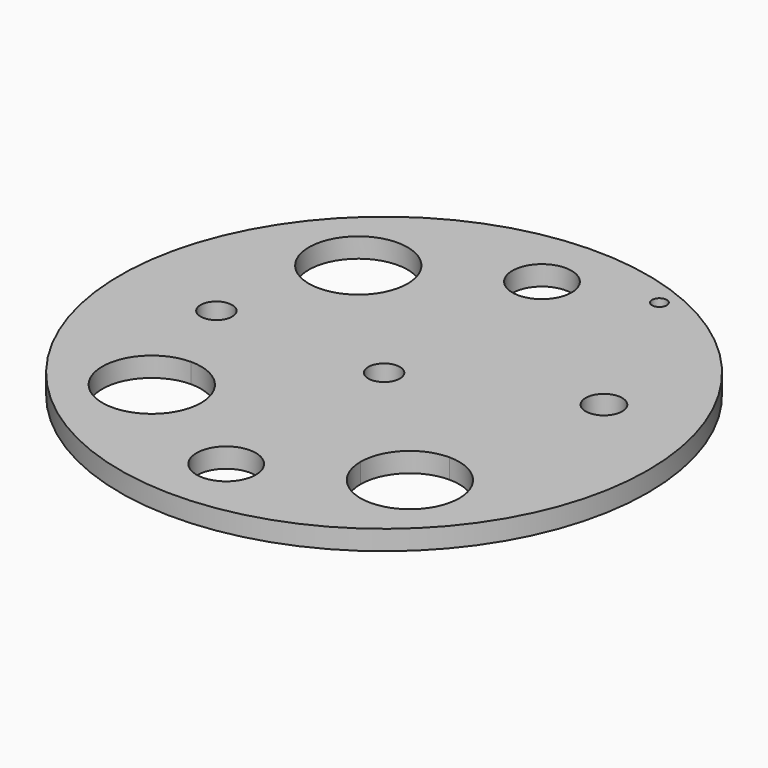
from build123d import *

# Parameters (mm, degrees)
F0_R     = 26.75
F0_R_2   = 3
F0_R_3   = 1.6
F0_R_4   = 1.85
F0_R_5   = 0.75
F1_DEPTH = 2


# Not quite as in the source:
# - a feature names something its author has since deleted; it is built from what else it names


with BuildPart() as f1:
    # F0 (on Top) → F1 (new body)
    with BuildSketch(Plane.XY):
        Circle(F0_R)
        with Locations((0, -20)):
            Circle(F0_R_2, mode=Mode.SUBTRACT)
        with Locations((-17, 0)):
            Circle(F0_R_3, mode=Mode.SUBTRACT)
        with BuildLine():
            Line((-8.081475452, 13.081475452), (13.081475452, 13.081475452))
            Line((13.081475452, 13.081475452), (13.081475452, -8.081475452))
            ThreePointArc((13.081475452, -8.081475452), (16.6170093579, -9.545941546), (18.081475452, -13.081475452))
            ThreePointArc((18.081475452, -13.081475452), (13.081475452, -18.081475452), (8.081475452, -13.081475452))
            Line((8.081475452, -13.081475452), (-8.081475452, -13.081475452))
            ThreePointArc((-8.081475452, -13.081475452), (-16.6170093579, -16.6170093579), (-13.081475452, -8.081475452))
            Line((-13.081475452, -8.081475452), (-13.081475452, 8.081475452))
            ThreePointArc((-13.081475452, 8.081475452), (-16.6170093579, 16.6170093579), (-8.081475452, 13.081475452))
        make_face(mode=Mode.SUBTRACT)
        with Locations((0, 20)):
            Circle(F0_R_2, mode=Mode.SUBTRACT)
        with Locations((17, 6.6)):
            Circle(F0_R_4, mode=Mode.SUBTRACT)
        with Locations((9.5, 23)):
            Circle(F0_R_5, mode=Mode.SUBTRACT)
        with BuildLine():
            Line((13.081475452, -8.081475452), (13.081475452, 13.081475452))
            Line((13.081475452, 13.081475452), (-8.081475452, 13.081475452))
            ThreePointArc((-8.081475452, 13.081475452), (-9.545941546, 9.545941546), (-13.081475452, 8.081475452))
            Line((-13.081475452, 8.081475452), (-13.081475452, -8.081475452))
            ThreePointArc((-13.081475452, -8.081475452), (-9.545941546, -9.545941546), (-8.081475452, -13.081475452))
            Line((-8.081475452, -13.081475452), (8.081475452, -13.081475452))
            ThreePointArc((8.081475452, -13.081475452), (9.545941546, -9.545941546), (13.081475452, -8.081475452))
        make_face()
        Circle(F0_R_3, mode=Mode.SUBTRACT)
    extrude(amount=F1_DEPTH)


solid = f1.part
